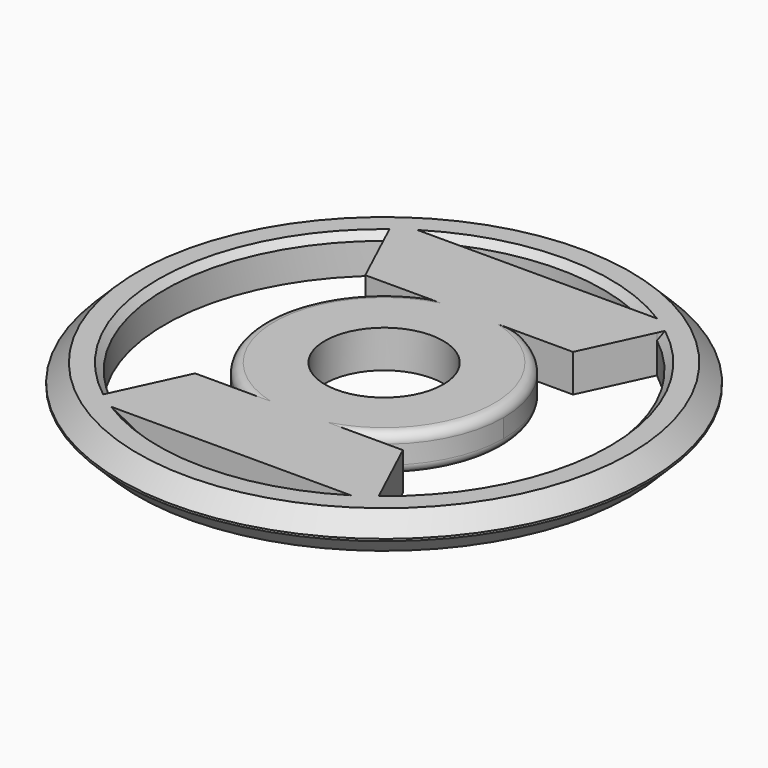
from build123d import *

# Parameters (mm, degrees)
F0_R         = 49.0432335283
F0_R_2       = 10.9855
F1_DEPTH     = 6.985
F2_T4_ANGLE  = 164.4789683114
F2_T10_ANGLE = 164.4789683114
F2_T16_ANGLE = 164.4789683114
F2_T22_ANGLE = 164.4789683114
F3_T4_ANGLE  = 113.2359316918
F3_T10_ANGLE = 67.3888483325
F3_T15_ANGLE = 113.2359316918
F3_T21_ANGLE = 67.3888483325
F4_SIZE      = 3.302


# Not quite as in the source:
# - a fillet or chamfer that OpenCascade refuses, or shapes differently, is made with other operations: its cross-section is extruded or revolved along the edge and cut away or added


with BuildPart() as f1:
    # F0 (on Top) → F1 (new body)
    with BuildSketch(Plane.XY):
        Circle(F0_R)
        with BuildLine():
            Line((26.67, 35.56), (25.0451862182, 32.0755756003))
            ThreePointArc((25.0451862182, 32.0755756003), (36.5740630803, 17.8449380104), (40.6952565147, 0))
            ThreePointArc((40.6952565147, 0), (36.5738989199, -17.8452744611), (25.0445960757, -32.0760363854))
            Line((25.0445960757, -32.0760363854), (26.67, -35.56))
            Line((26.67, -35.56), (19.7886407516, -35.56))
            ThreePointArc((19.7886407516, -35.56), (0, -40.6952565147), (-19.7886407516, -35.56))
            Line((-19.7886407516, -35.56), (-26.67, -35.56))
            Line((-26.67, -35.56), (-25.0445960757, -32.0760363854))
            ThreePointArc((-25.0445960757, -32.0760363854), (-40.695256513, -0.0003743631), (-25.0451862182, 32.0755756003))
            Line((-25.0451862182, 32.0755756003), (-26.67, 35.56))
            Line((-26.67, 35.56), (-19.7886407516, 35.56))
            ThreePointArc((-19.7886407516, 35.56), (0, 40.6952565147), (19.7886407516, 35.56))
            Line((19.7886407516, 35.56), (26.67, 35.56))
        make_face(mode=Mode.SUBTRACT)
        with BuildLine():
            ThreePointArc((-10.1860168797, 19.7533714876), (0, 22.225), (10.1860168797, 19.7533714876))
            Line((10.1860168797, 19.7533714876), (19.299248075, 19.7533714876))
            Line((19.299248075, 19.7533714876), (25.0451862182, 32.0755756003))
            ThreePointArc((25.0451862182, 32.0755756003), (22.4845127485, 33.9197669399), (19.7886407516, 35.56))
            Line((19.7886407516, 35.56), (-19.7886407516, 35.56))
            ThreePointArc((-19.7886407516, 35.56), (-22.4845127485, 33.9197669399), (-25.0451862182, 32.0755756003))
            Line((-25.0451862182, 32.0755756003), (-19.299248075, 19.7533714876))
            Line((-19.299248075, 19.7533714876), (-10.1860168797, 19.7533714876))
        make_face()
        with BuildLine():
            Line((-26.67, 35.56), (-25.0451862182, 32.0755756003))
            ThreePointArc((-25.0451862182, 32.0755756003), (-22.4845127485, 33.9197669399), (-19.7886407516, 35.56))
            Line((-19.7886407516, 35.56), (-26.67, 35.56))
        make_face()
        with BuildLine():
            ThreePointArc((19.7886407516, 35.56), (22.4845127485, 33.9197669399), (25.0451862182, 32.0755756003))
            Line((25.0451862182, 32.0755756003), (26.67, 35.56))
            Line((26.67, 35.56), (19.7886407516, 35.56))
        make_face()
        with BuildLine():
            ThreePointArc((10.1708209875, -19.7612), (18.9736280327, -11.5737662097), (22.225, 0))
            ThreePointArc((22.225, 0), (18.9780774863, 11.5664687751), (10.1860168797, 19.7533714876))
            Line((10.1860168797, 19.7533714876), (0, 19.7533714876))
            Line((0, 19.7533714876), (-10.1860168797, 19.7533714876))
            ThreePointArc((-10.1860168797, 19.7533714876), (-22.2249983566, -0.0085469402), (-10.1708209875, -19.7612))
            Line((-10.1708209875, -19.7612), (0, -19.7612))
            Line((0, -19.7612), (10.1708209875, -19.7612))
        make_face()
        Circle(F0_R_2, mode=Mode.SUBTRACT)
        with BuildLine():
            Line((0, 19.7533714876), (10.1860168797, 19.7533714876))
            ThreePointArc((10.1860168797, 19.7533714876), (0, 22.225), (-10.1860168797, 19.7533714876))
            Line((-10.1860168797, 19.7533714876), (0, 19.7533714876))
        make_face()
        with BuildLine():
            Line((19.299248075, -19.7612), (10.1708209875, -19.7612))
            ThreePointArc((10.1708209875, -19.7612), (0, -22.225), (-10.1708209875, -19.7612))
            Line((-10.1708209875, -19.7612), (-19.299248075, -19.7612))
            Line((-19.299248075, -19.7612), (-25.0445960757, -32.0760363854))
            ThreePointArc((-25.0445960757, -32.0760363854), (-22.4842007134, -33.9199737776), (-19.7886407516, -35.56))
            Line((-19.7886407516, -35.56), (19.7886407516, -35.56))
            ThreePointArc((19.7886407516, -35.56), (22.4842007134, -33.9199737776), (25.0445960757, -32.0760363854))
            Line((25.0445960757, -32.0760363854), (19.299248075, -19.7612))
        make_face()
        with BuildLine():
            ThreePointArc((-10.1708209875, -19.7612), (0, -22.225), (10.1708209875, -19.7612))
            Line((10.1708209875, -19.7612), (0, -19.7612))
            Line((0, -19.7612), (-10.1708209875, -19.7612))
        make_face()
        with BuildLine():
            ThreePointArc((-19.7886407516, -35.56), (-22.4842007134, -33.9199737776), (-25.0445960757, -32.0760363854))
            Line((-25.0445960757, -32.0760363854), (-26.67, -35.56))
            Line((-26.67, -35.56), (-19.7886407516, -35.56))
        make_face()
        with BuildLine():
            Line((26.67, -35.56), (25.0445960757, -32.0760363854))
            ThreePointArc((25.0445960757, -32.0760363854), (22.4842007134, -33.9199737776), (19.7886407516, -35.56))
            Line((19.7886407516, -35.56), (26.67, -35.56))
        make_face()
    extrude(amount=F1_DEPTH)

    # F2: fillet of radius 1.778 on 4 edges, made by hand


with BuildPart() as f2_tool2:
    # F2_s3 → F2_t4 (revolve)
    with BuildSketch(Plane(origin=(0, 0, 0), x_dir=(0, 0, 1), z_dir=(0.9907891286, 0.1354138197, 0))):
        with BuildLine():
            ThreePointArc((5.207, -22.225), (6.4642358569, -21.7042358569), (6.985, -20.447))
            Line((6.985, -20.447), (6.985, -22.225))
            Line((6.985, -22.225), (5.207, -22.225))
        make_face()
    revolve(axis=Axis((0, 0, 6.985), (0, 0, 1)), revolution_arc=F2_T4_ANGLE)

    split(bisect_by=Plane.XZ.offset(-19.7533714876), keep=Keep.TOP)

    split(bisect_by=Plane.XZ.offset(19.7612), keep=Keep.BOTTOM)


with BuildPart() as f1_1:
    add(f1.part)

    # F2_t1: cut F2_tool2
    add(f2_tool2.part, mode=Mode.SUBTRACT)


with BuildPart() as f2_tool8:
    # F2_s9 → F2_t10 (revolve)
    with BuildSketch(Plane(origin=(0, 0, 0), x_dir=(0, 0, 1), z_dir=(-0.9908929862, -0.1346517356, 0))):
        with BuildLine():
            ThreePointArc((5.207, -22.225), (6.4642358569, -21.7042358569), (6.985, -20.447))
            Line((6.985, -20.447), (6.985, -22.225))
            Line((6.985, -22.225), (5.207, -22.225))
        make_face()
    revolve(axis=Axis((0, 0, 6.985), (0, 0, 1)), revolution_arc=F2_T10_ANGLE)

    split(bisect_by=Plane.XZ.offset(19.7612), keep=Keep.BOTTOM)

    split(bisect_by=Plane.XZ.offset(-19.7533714876), keep=Keep.TOP)


with BuildPart() as f1_2:
    add(f1_1.part)

    # F2_t7: cut F2_tool8
    add(f2_tool8.part, mode=Mode.SUBTRACT)


with BuildPart() as f2_tool14:
    # F2_s15 → F2_t16 (revolve)
    with BuildSketch(Plane(origin=(0, 0, 0), x_dir=(0, 0, 1), z_dir=(-0.9908929862, -0.1346517356, 0))):
        with BuildLine():
            ThreePointArc((1.778, -22.225), (0.5207641431, -21.7042358569), (0, -20.447))
            Line((0, -20.447), (0, -22.225))
            Line((0, -22.225), (1.778, -22.225))
        make_face()
    revolve(axis=Axis((0, 0, 0), (0, 0, 1)), revolution_arc=F2_T16_ANGLE)

    split(bisect_by=Plane.XZ.offset(19.7612), keep=Keep.BOTTOM)

    split(bisect_by=Plane.XZ.offset(-19.7533714876), keep=Keep.TOP)


with BuildPart() as f1_3:
    add(f1_2.part)

    # F2_t13: cut F2_tool14
    add(f2_tool14.part, mode=Mode.SUBTRACT)


with BuildPart() as f2_tool20:
    # F2_s21 → F2_t22 (revolve)
    with BuildSketch(Plane(origin=(0, 0, 0), x_dir=(0, 0, 1), z_dir=(0.9907891286, 0.1354138197, 0))):
        with BuildLine():
            ThreePointArc((1.778, -22.225), (0.5207641431, -21.7042358569), (0, -20.447))
            Line((0, -20.447), (0, -22.225))
            Line((0, -22.225), (1.778, -22.225))
        make_face()
    revolve(axis=Axis((0, 0, 0), (0, 0, 1)), revolution_arc=F2_T22_ANGLE)

    split(bisect_by=Plane.XZ.offset(-19.7533714876), keep=Keep.TOP)

    split(bisect_by=Plane.XZ.offset(19.7612), keep=Keep.BOTTOM)


with BuildPart() as f1_4:
    add(f1_3.part)

    # F2_t19: cut F2_tool20
    add(f2_tool20.part, mode=Mode.SUBTRACT)

    # F3: chamfer of 1.27 on 4 edges, made by hand


with BuildPart() as f3_tool2:
    # F3_s3 → F3_t4 (revolve)
    with BuildSketch(Plane(origin=(0, 0, 0), x_dir=(0, 0, 1), z_dir=(0.8350254942, -0.550211254, 0))):
        Polygon((6.985, 41.9652565147), (5.715, 40.6952565147), (6.985, 40.6952565147), align=None)
    revolve(axis=Axis((0, 0, 6.985), (0, 0, -1)), revolution_arc=F3_T4_ANGLE)

    split(bisect_by=Plane(origin=(-8.2863025765, -3.8639663492, 0), x_dir=(0, 0, 1), z_dir=(-0.906307787, -0.4226182617, 0)), keep=Keep.TOP)

    split(bisect_by=Plane(origin=(-8.2780879413, 3.8620485498, 0), x_dir=(0, 0, 1), z_dir=(-0.906227568, 0.4227902494, 0)), keep=Keep.TOP)


with BuildPart() as f1_5:
    add(f1_4.part)

    # F3_t1: cut F3_tool2
    add(f3_tool2.part, mode=Mode.SUBTRACT)


with BuildPart() as f3_tool8:
    # F3_s9 → F3_t10 (revolve)
    with BuildSketch(Plane(origin=(0, 0, 0), x_dir=(0, 0, 1), z_dir=(-0.8320081138, -0.5547634618, 0))):
        Polygon((6.985, 41.9652565147), (5.715, 40.6952565147), (6.985, 40.6952565147), align=None)
    revolve(axis=Axis((0, 0, 6.985), (0, 0, -1)), revolution_arc=F3_T10_ANGLE)

    split(bisect_by=Plane.XZ.offset(-35.56), keep=Keep.BOTTOM)


with BuildPart() as f1_6:
    add(f1_5.part)

    # F3_t7: cut F3_tool8
    add(f3_tool8.part, mode=Mode.SUBTRACT)


with BuildPart() as f3_tool13:
    # F3_s14 → F3_t15 (revolve)
    with BuildSketch(Plane(origin=(0, 0, 0), x_dir=(0, 0, 1), z_dir=(-0.8350153711, 0.550226617, 0))):
        Polygon((6.985, 41.9652565147), (5.715, 40.6952565147), (6.985, 40.6952565147), align=None)
    revolve(axis=Axis((0, 0, 6.985), (0, 0, -1)), revolution_arc=F3_T15_ANGLE)

    split(bisect_by=Plane(origin=(8.2780879413, 3.8620485498, 0), x_dir=(0, 0, 1), z_dir=(0.906227568, 0.4227902494, 0)), keep=Keep.TOP)

    split(bisect_by=Plane(origin=(8.2863025765, -3.8639663492, 0), x_dir=(0, 0, 1), z_dir=(0.906307787, -0.4226182617, 0)), keep=Keep.TOP)


with BuildPart() as f1_7:
    add(f1_6.part)

    # F3_t12: cut F3_tool13
    add(f3_tool13.part, mode=Mode.SUBTRACT)


with BuildPart() as f3_tool19:
    # F3_s20 → F3_t21 (revolve)
    with BuildSketch(Plane(origin=(0, 0, 0), x_dir=(0, 0, 1), z_dir=(0.8320081138, 0.5547634618, 0))):
        Polygon((6.985, 41.9652565147), (5.715, 40.6952565147), (6.985, 40.6952565147), align=None)
    revolve(axis=Axis((0, 0, 6.985), (0, 0, -1)), revolution_arc=F3_T21_ANGLE)

    split(bisect_by=Plane.XZ.offset(35.56), keep=Keep.TOP)


with BuildPart() as f1_8:
    add(f1_7.part)

    # F3_t18: cut F3_tool19
    add(f3_tool19.part, mode=Mode.SUBTRACT)

    # F4
    f4_edges = [f1_8.edges().sort_by_distance(p)[0] for p in [
        (-49.043234, 0, 6.985),
        (-49.043234, 0, 0),
    ]]
    chamfer(f4_edges, length=F4_SIZE)


solid = f1_8.part
